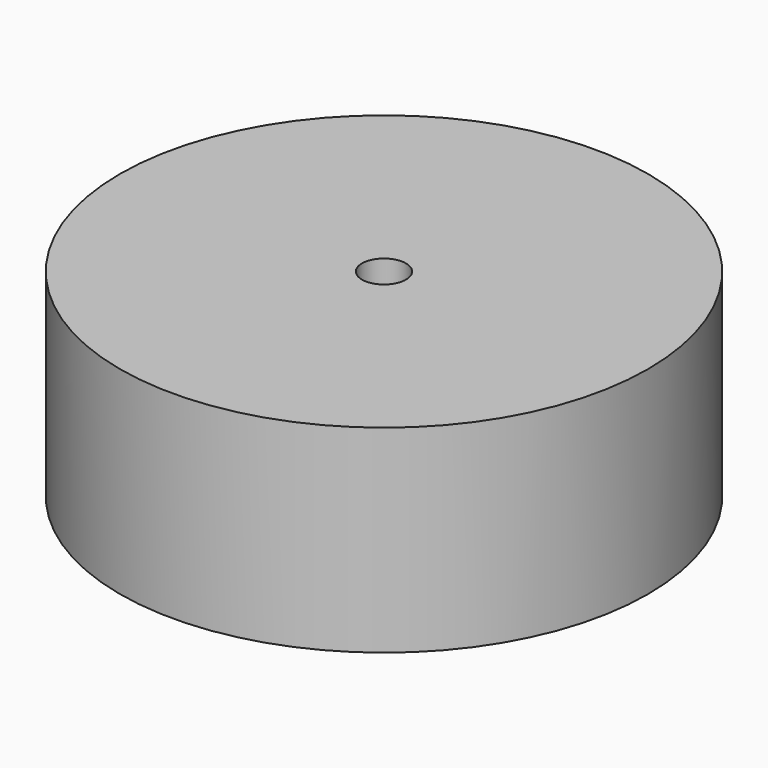
from build123d import *

# Parameters (mm, degrees)
F0_R     = 76.2
F1_DEPTH = 57.15
F4_D     = 12.7


# Not quite as in the source:
# - a length typed as a fraction of an inch, garbled in the dataset ("3 / 203.2 mm" for 3/8 in), is restored


with BuildPart() as f1:
    # F0 (on Top) → F1 (new body)
    with BuildSketch(Plane.XY):
        Circle(F0_R)
    extrude(amount=F1_DEPTH)

    # F4 (through all)
    with Locations(Plane.XY.offset(57.15)):
        with Locations((510.4262828827, -143.8676267862), (0, 0)):
            Hole(F4_D / 2)


solid = f1.part
